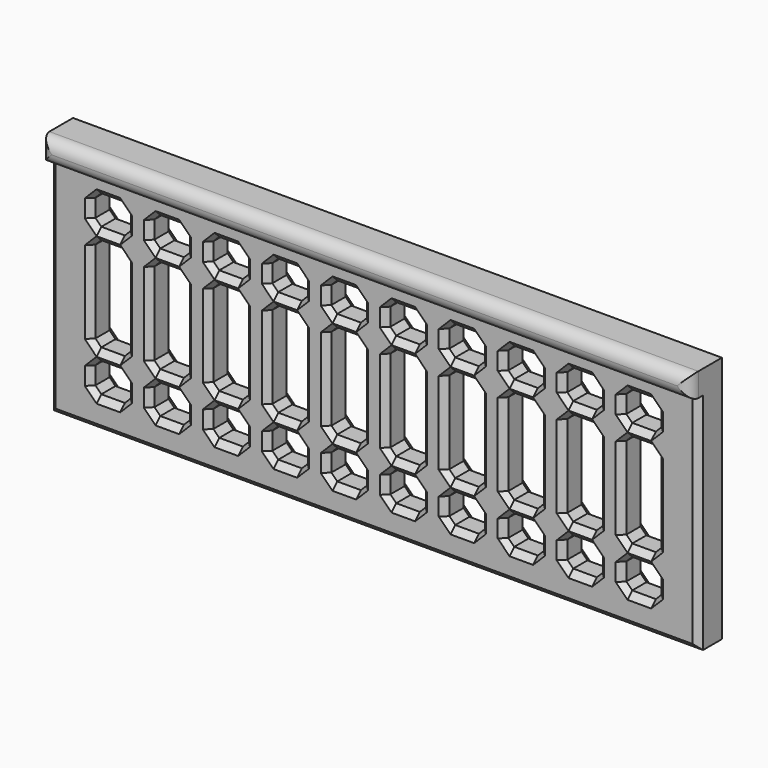
from build123d import *

# Parameters (mm, degrees)
F0_W     = 110
F0_H     = 40
F0_W_2   = 106
F0_H_2   = 34
F0_W_3   = 4
F0_H_3   = 16
F0_W_4   = 6
F0_H_4   = 2
F1_DEPTH = 5
F2_SIZE  = 0.99999
F3_W     = 7
F3_H     = 4
F4_DEPTH = 110
F5_R     = 1.99999


# Not quite as in the source:
# - a fillet or chamfer is up to 0.001 mm smaller than in the source, because OpenCascade refuses the exact size
# - a feature names something its author has since deleted; it is built from what else it names


with BuildPart() as f1:
    # F0 (on Front) → F1 (new body)
    with BuildSketch(Plane.XZ):
        with Locations((55, 20)):
            Rectangle(F0_W, F0_H)
        with Locations((55, 20)):
            Rectangle(F0_W_2, F0_H_2, mode=Mode.SUBTRACT)
        with Locations((55, 20)):
            Rectangle(F0_W_2, F0_H_2)
        Polygon((7, 30), (7, 35), (13, 35), (13, 30), (17, 30), (17, 35), (23, 35), (23, 30), (27, 30), (27, 35), (33, 35), (33, 30), (37, 30), (37, 35), (43, 35), (43, 30), (47, 30), (47, 35), (53, 35), (53, 30), (57, 30), (57, 35), (63, 35), (63, 30), (67, 30), (67, 35), (73, 35), (73, 30), (77, 30), (77, 35), (83, 35), (83, 30), (87, 30), (87, 35), (93, 35), (93, 30), (97, 30), (97, 35), (103, 35), (103, 30), (103, 28), (103, 12), (103, 10), (103, 5), (97, 5), (97, 10), (93, 10), (93, 5), (87, 5), (87, 10), (83, 10), (83, 5), (77, 5), (77, 10), (73, 10), (73, 5), (67, 5), (67, 10), (63, 10), (63, 5), (57, 5), (57, 10), (53, 10), (53, 5), (47, 5), (47, 10), (43, 10), (43, 5), (37, 5), (37, 10), (33, 10), (33, 5), (27, 5), (27, 10), (23, 10), (23, 5), (17, 5), (17, 10), (13, 10), (13, 5), (7, 5), (7, 10), (7, 12), (7, 28), align=None, mode=Mode.SUBTRACT)
        with Locations((25, 20)):
            Rectangle(F0_W_3, F0_H_3)
        with Locations((15, 20)):
            Rectangle(F0_W_3, F0_H_3)
        with Locations((35, 20)):
            Rectangle(F0_W_3, F0_H_3)
        with Locations((45, 20)):
            Rectangle(F0_W_3, F0_H_3)
        with Locations((85, 20)):
            Rectangle(F0_W_3, F0_H_3)
        with Locations((95, 20)):
            Rectangle(F0_W_3, F0_H_3)
        with Locations((55, 20)):
            Rectangle(F0_W_3, F0_H_3)
        with Locations((65, 20)):
            Rectangle(F0_W_3, F0_H_3)
        with Locations((75, 20)):
            Rectangle(F0_W_3, F0_H_3)
        with Locations((10, 29)):
            Rectangle(F0_W_4, F0_H_4)
        with Locations((10, 11)):
            Rectangle(F0_W_4, F0_H_4)
        with Locations((20, 11)):
            Rectangle(F0_W_4, F0_H_4)
        with Locations((20, 29)):
            Rectangle(F0_W_4, F0_H_4)
        with Locations((30, 11)):
            Rectangle(F0_W_4, F0_H_4)
        with Locations((30, 29)):
            Rectangle(F0_W_4, F0_H_4)
        with Locations((40, 29)):
            Rectangle(F0_W_4, F0_H_4)
        with Locations((40, 11)):
            Rectangle(F0_W_4, F0_H_4)
        with Locations((50, 11)):
            Rectangle(F0_W_4, F0_H_4)
        with Locations((50, 29)):
            Rectangle(F0_W_4, F0_H_4)
        with Locations((80, 29)):
            Rectangle(F0_W_4, F0_H_4)
        with Locations((80, 11)):
            Rectangle(F0_W_4, F0_H_4)
        with Locations((90, 11)):
            Rectangle(F0_W_4, F0_H_4)
        with Locations((90, 29)):
            Rectangle(F0_W_4, F0_H_4)
        with Locations((100, 29)):
            Rectangle(F0_W_4, F0_H_4)
        with Locations((100, 11)):
            Rectangle(F0_W_4, F0_H_4)
        with Locations((60, 29)):
            Rectangle(F0_W_4, F0_H_4)
        with Locations((60, 11)):
            Rectangle(F0_W_4, F0_H_4)
        with Locations((70, 11)):
            Rectangle(F0_W_4, F0_H_4)
        with Locations((70, 29)):
            Rectangle(F0_W_4, F0_H_4)
        with Locations((15, 29)):
            Rectangle(F0_W_3, F0_H_4)
        with Locations((15, 11)):
            Rectangle(F0_W_3, F0_H_4)
        with Locations((25, 11)):
            Rectangle(F0_W_3, F0_H_4)
        with Locations((25, 29)):
            Rectangle(F0_W_3, F0_H_4)
        with Locations((35, 11)):
            Rectangle(F0_W_3, F0_H_4)
        with Locations((35, 29)):
            Rectangle(F0_W_3, F0_H_4)
        with Locations((45, 29)):
            Rectangle(F0_W_3, F0_H_4)
        with Locations((45, 11)):
            Rectangle(F0_W_3, F0_H_4)
        with Locations((85, 29)):
            Rectangle(F0_W_3, F0_H_4)
        with Locations((85, 11)):
            Rectangle(F0_W_3, F0_H_4)
        with Locations((95, 29)):
            Rectangle(F0_W_3, F0_H_4)
        with Locations((95, 11)):
            Rectangle(F0_W_3, F0_H_4)
        with Locations((55, 29)):
            Rectangle(F0_W_3, F0_H_4)
        with Locations((55, 11)):
            Rectangle(F0_W_3, F0_H_4)
        with Locations((65, 11)):
            Rectangle(F0_W_3, F0_H_4)
        with Locations((75, 11)):
            Rectangle(F0_W_3, F0_H_4)
        with Locations((65, 29)):
            Rectangle(F0_W_3, F0_H_4)
        with Locations((75, 29)):
            Rectangle(F0_W_3, F0_H_4)
    extrude(amount=F1_DEPTH)

    # F2 (size 1 in the source; OpenCascade refuses exactly that, so slightly less here)
    f2_edges = [f1.edges().sort_by_distance(p)[0] for p in [
        (47, 0, 32.5),
        (60, 0, 28),
        (50, 0, 28),
        (50, -5, 28),
        (47, -5, 20),
        (50, -5, 12),
        (53, -5, 20),
        (50, -5, 30),
        (53, -5, 32.5),
        (50, -5, 35),
        (47, -5, 32.5),
        (50, -5, 10),
        (53, -5, 7.5),
        (50, -5, 5),
        (47, -5, 7.5),
        (43, -5, 7.5),
        (37, -5, 7.5),
        (40, -5, 10),
        (40, -5, 5),
        (40, -5, 12),
        (43, -5, 20),
        (37, -5, 20),
        (40, -5, 28),
        (40, -5, 30),
        (33, -5, 7.5),
        (30, -5, 5),
        (27, -5, 7.5),
        (30, -5, 10),
        (30, -5, 12),
        (33, -5, 20),
        (27, -5, 20),
        (30, -5, 28),
        (30, -5, 30),
        (110, -5, 20),
        (55, -5, 40),
        (0, -5, 20),
        (55, -5, 0),
        (20, -5, 12),
        (83, -2.5, 28),
        (63, -5, 7.5),
        (17, -5, 7.5),
        (7, -5, 32.5),
        (17, -5, 20),
        (20, -5, 5),
        (57, -2.5, 10),
        (60, -5, 10),
        (87, -5, 20),
        (77, -5, 32.5),
        (57, -5, 7.5),
        (100, -5, 35),
        (43, -5, 32.5),
        (30, -5, 35),
        (23, -5, 20),
        (80, -5, 10),
        (70, -5, 5),
        (80, -5, 28),
        (73, -5, 7.5),
        (23, -2.5, 12),
        (83, -5, 32.5),
        (70, -5, 30),
        (27, -5, 32.5),
        (67, -5, 20),
        (13, -5, 20),
        (93, -5, 20),
        (80, -5, 12),
        (17, -5, 32.5),
        (93, -5, 32.5),
        (33, -5, 32.5),
        (20, -5, 28),
        (93, -5, 7.5),
        (10, -5, 28),
        (13, -5, 7.5),
        (43, -2.5, 12),
        (83, -2.5, 30),
        (87, -5, 7.5),
        (103, -5, 7.5),
        (103, -5, 20),
        (90, -5, 30),
        (23, -5, 7.5),
        (87, -5, 32.5),
        (67, -5, 32.5),
        (97, -5, 7.5),
        (80, -5, 30),
        (43, -2.5, 28),
        (63, -5, 32.5),
        (10, -5, 5),
        (70, -5, 10),
        (7, -5, 7.5),
        (37, -5, 32.5),
        (77, -5, 7.5),
        (70, -5, 28),
        (77, -5, 20),
        (60, -5, 28),
        (73, -5, 20),
        (67, -5, 7.5),
        (83, -2.5, 12),
        (83, -5, 20),
        (60, -5, 30),
        (90, -5, 28),
        (97, -5, 32.5),
        (100, -5, 5),
        (70, -5, 12),
        (57, -5, 32.5),
        (57, -5, 20),
        (43, -2.5, 10),
        (90, -5, 35),
        (10, -5, 35),
        (33, -2.5, 28),
        (73, -5, 32.5),
        (80, -5, 35),
        (7, -5, 20),
        (23, -2.5, 30),
        (10, -5, 10),
        (60, -5, 35),
        (70, -5, 35),
        (63, -5, 20),
        (20, -5, 35),
        (80, -5, 5),
        (20, -5, 30),
        (13, -5, 32.5),
        (90, -5, 10),
        (100, -5, 30),
        (100, -5, 10),
        (90, -5, 5),
        (20, -5, 10),
        (83, -5, 7.5),
        (90, -5, 12),
        (23, -5, 32.5),
        (97, -5, 20),
        (60, -5, 5),
        (100, -5, 12),
        (80, 0, 10),
        (33, 0, 7.5),
        (37, 0, 7.5),
        (87, -2.5, 30),
        (7, -2.5, 10),
        (23, -2.5, 35),
        (87, -2.5, 28),
        (97, -2.5, 5),
        (50, 0, 35),
        (17, 0, 32.5),
        (103, -2.5, 12),
        (33, -2.5, 5),
        (10, 0, 35),
        (60, 0, 30),
        (37, -2.5, 12),
        (47, -2.5, 28),
        (17, -2.5, 10),
        (20, 0, 28),
        (70, 0, 28),
        (70, 0, 12),
        (80, 0, 28),
        (63, -2.5, 30),
        (100, 0, 5),
        (23, -2.5, 5),
        (100, 0, 10),
        (63, 0, 20),
        (80, 0, 5),
        (20, 0, 35),
        (93, -2.5, 35),
        (93, -2.5, 10),
        (83, -2.5, 10),
        (57, 0, 20),
        (37, 0, 20),
        (90, 0, 28),
        (73, -2.5, 10),
        (53, -2.5, 28),
        (87, -2.5, 10),
        (87, -2.5, 12),
        (93, -2.5, 28),
        (97, 0, 20),
        (17, 0, 7.5),
        (43, -2.5, 30),
        (80, 0, 35),
        (7, 0, 32.5),
        (43, -2.5, 35),
        (67, 0, 20),
        (97, -2.5, 12),
        (67, -2.5, 28),
        (13, -2.5, 35),
        (40, 0, 12),
        (27, -2.5, 5),
        (70, 0, 5),
        (77, -2.5, 30),
        (87, 0, 32.5),
        (13, -2.5, 10),
        (13, 0, 20),
        (93, -2.5, 12),
        (77, 0, 7.5),
        (33, -2.5, 30),
        (77, -2.5, 10),
        (100, -5, 28),
        (30, 0, 10),
        (47, 0, 20),
        (47, -2.5, 10),
        (10, 0, 28),
        (17, -2.5, 5),
        (43, 0, 7.5),
        (23, 0, 20),
        (13, 0, 32.5),
        (17, -2.5, 12),
        (103, -2.5, 10),
        (73, 0, 32.5),
        (100, 0, 30),
        (33, 0, 20),
        (63, -2.5, 28),
        (93, 0, 32.5),
        (40, -5, 35),
        (7, 0, 20),
        (57, 0, 7.5),
        (57, -2.5, 5),
        (17, 0, 20),
        (67, -2.5, 12),
        (90, 0, 30),
        (43, -2.5, 5),
        (33, 0, 32.5),
        (43, 0, 20),
        (87, 0, 7.5),
        (63, 0, 32.5),
        (70, 0, 10),
        (23, 0, 7.5),
        (73, -2.5, 5),
        (7, -2.5, 35),
        (30, 0, 5),
        (67, -2.5, 10),
        (67, 0, 7.5),
        (43, 0, 32.5),
        (17, -2.5, 28),
        (33, -2.5, 35),
        (70, 0, 30),
        (37, -2.5, 35),
        (10, 0, 5),
        (87, 0, 20),
        (20, 0, 10),
        (67, -2.5, 5),
        (10, 0, 10),
        (67, 0, 32.5),
        (93, 0, 20),
        (60, 0, 10),
        (97, -2.5, 30),
        (63, -2.5, 5),
        (87, -2.5, 35),
        (40, 0, 30),
        (63, -2.5, 10),
        (23, -2.5, 28),
        (70, 0, 35),
        (90, 0, 5),
        (20, 0, 12),
        (27, -2.5, 10),
        (100, 0, 35),
        (80, 0, 30),
        (67, -2.5, 30),
        (27, -2.5, 12),
        (77, 0, 20),
        (47, -2.5, 12),
        (57, -2.5, 28),
        (40, 0, 5),
        (57, -2.5, 35),
        (37, -2.5, 30),
        (27, -2.5, 28),
        (73, -2.5, 30),
        (93, -2.5, 30),
        (73, -2.5, 35),
        (73, -2.5, 28),
        (103, -5, 32.5),
        (57, -2.5, 30),
        (90, 0, 35),
        (7, 0, 7.5),
        (20, 0, 30),
        (47, -2.5, 30),
        (83, -2.5, 5),
        (30, 0, 35),
        (73, 0, 7.5),
        (30, 0, 30),
        (73, 0, 20),
        (83, -2.5, 35),
        (83, 0, 7.5),
        (63, 0, 7.5),
        (27, 0, 32.5),
        (27, -2.5, 35),
        (37, -2.5, 28),
        (33, -2.5, 12),
        (60, 0, 5),
        (17, -2.5, 30),
        (33, -2.5, 10),
        (47, -2.5, 5),
        (97, -2.5, 35),
        (60, -5, 12),
        (103, 0, 20),
        (13, -2.5, 5),
        (83, 0, 32.5),
        (30, 0, 12),
        (97, 0, 32.5),
        (27, 0, 20),
        (77, -2.5, 12),
        (27, 0, 7.5),
        (90, 0, 12),
        (77, -2.5, 5),
        (57, 0, 32.5),
        (103, 0, 7.5),
        (60, 0, 35),
        (47, 0, 7.5),
        (20, 0, 5),
        (53, -2.5, 12),
        (13, -2.5, 28),
        (77, -2.5, 35),
        (103, -2.5, 30),
        (67, -2.5, 35),
        (23, -2.5, 10),
        (7, -2.5, 28),
        (47, -2.5, 35),
        (97, -2.5, 28),
        (27, -2.5, 30),
        (30, 0, 28),
        (10, -5, 12),
        (97, 0, 7.5),
        (77, -2.5, 28),
        (23, 0, 32.5),
        (63, -2.5, 35),
        (37, -2.5, 5),
        (90, 0, 10),
        (77, 0, 32.5),
        (37, 0, 32.5),
        (97, -2.5, 10),
        (93, -2.5, 5),
        (17, -2.5, 35),
        (13, 0, 7.5),
        (80, 0, 12),
        (7, -2.5, 5),
        (53, -2.5, 35),
        (50, 0, 12),
        (103, -2.5, 5),
        (73, -2.5, 12),
        (83, 0, 20),
        (53, 0, 32.5),
        (87, -2.5, 5),
        (93, 0, 7.5),
        (10, -5, 30),
        (40, 0, 10),
        (50, 0, 10),
        (53, 0, 7.5),
        (100, 0, 28),
        (40, 0, 28),
        (103, -2.5, 35),
        (53, -2.5, 10),
        (13, -2.5, 30),
        (50, 0, 5),
        (7, -2.5, 12),
        (13, -2.5, 12),
        (103, -2.5, 28),
        (103, 0, 32.5),
        (100, 0, 12),
        (7, -2.5, 30),
        (53, 0, 20),
        (63, -2.5, 12),
        (60, 0, 12),
        (37, -2.5, 10),
        (50, 0, 30),
        (53, -2.5, 30),
        (10, 0, 30),
        (57, -2.5, 12),
        (40, 0, 35),
        (10, 0, 12),
        (53, -2.5, 5),
    ]]
    chamfer(f2_edges, length=F2_SIZE)

    # F3 (on Right) → F4 (join)
    with BuildSketch(Plane.YZ):
        with Locations((-3.5, 40)):
            Rectangle(F3_W, F3_H)
    extrude(amount=F4_DEPTH)

    # F5 (radius 2 in the source; OpenCascade refuses exactly that, so slightly less here)
    f5_edges = [f1.edges().sort_by_distance(p)[0] for p in [
        (55, -7, 38),
        (55, -7, 42),
        (0, -7, 40),
        (110, -7, 40),
    ]]
    fillet(f5_edges, radius=F5_R)


solid = f1.part
